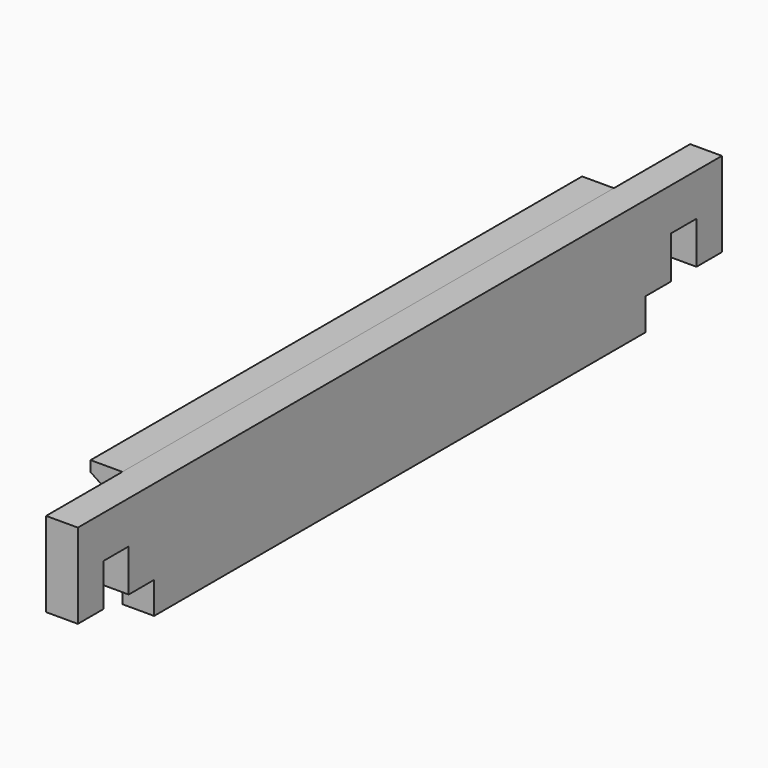
from build123d import *

# Parameters (mm, degrees)
F0_W          = 38.1
F0_H          = 482.6
F1_DEPTH      = 139.7
F2_W          = 114.3
F2_H          = 38.1
F3_DEPTH      = 38.101
F4_W          = 38.1
F4_H          = 50.8
F5_DEPTH      = 38.101
F9_DEPTH      = 368.3
F9_DEPTH_BACK = 368.3


# Not quite as in the source:
# - a feature names something its author has since deleted; it is built from what else it names


with BuildPart() as f1:
    # F0 (on Top) → F1 (new body)
    with BuildSketch(Plane.XY):
        with Locations((0, 241.3)):
            Rectangle(F0_W, F0_H)
    extrude(amount=-F1_DEPTH)

    # F2 (on face) → F3 (cut, through all)
    with BuildSketch(Plane.YZ.offset(19.05)):
        with Locations((57.15, -120.65)):
            Rectangle(F2_W, F2_H)
    extrude(amount=-F3_DEPTH, mode=Mode.SUBTRACT)

    # F4 (on face) → F5 (cut, through all)
    with BuildSketch(Plane.YZ.offset(19.05)):
        with Locations((57.15, -76.2)):
            Rectangle(F4_W, F4_H)
    extrude(amount=-F5_DEPTH, mode=Mode.SUBTRACT)

    # F7: F1 across plane


with BuildPart() as f1_1:
    add(f1.part)
    add(f1.part.mirror(Plane(origin=(0, 482.6, -69.85), x_dir=(-1, 0, 0), z_dir=(0, 1, 0))))


with BuildPart() as f9:
    # F8 (on offset) → F9 (new body, two sides)
    with BuildSketch(Plane(origin=(0, 482.6, 0), x_dir=(-1, 0, 0), z_dir=(0, 1, 0))) as f9_sk:
        Polygon((57.15, -12.7), (57.15, 0), (19.05, 0), (19.05, -38.1), align=None)
    extrude(amount=F9_DEPTH)
    extrude(f9_sk.sketch, amount=-F9_DEPTH_BACK)


solid = Compound([f1_1.part, f9.part])
